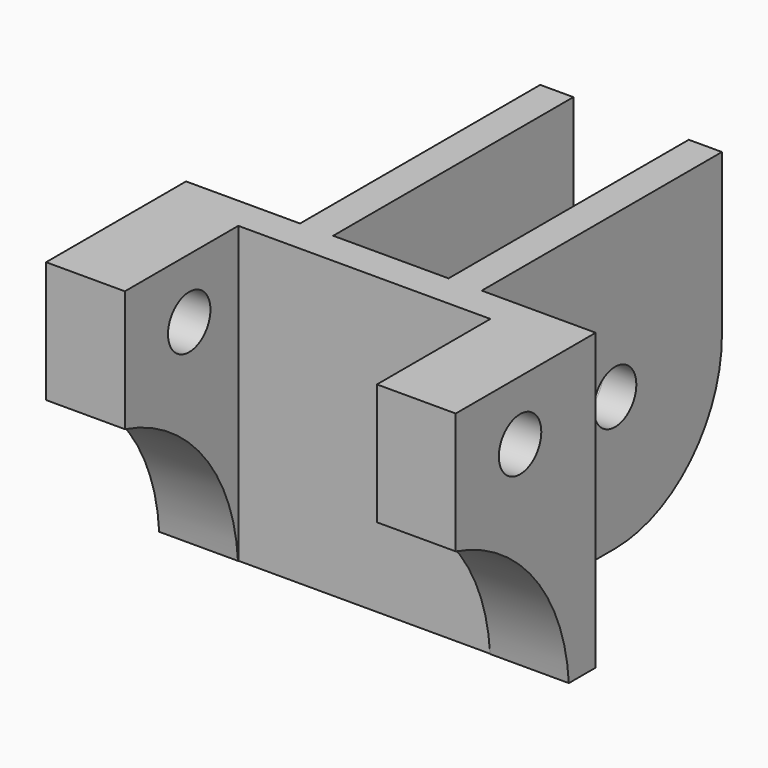
from build123d import *
from build123d import SkipClean  # not in build123d's __all__

# Parameters (mm, degrees)
F1_DEPTH  = 17.7784
F3_DEPTH  = 24.701
F4_R      = 1.6
F5_DEPTH  = 17.8292
F6_R      = 1.6
F7_DEPTH  = 24.701
F9_DEPTH  = 2
F10_R     = 3.2274
F10_R_2   = 1.6
F11_DEPTH = 0.5
F13_SIZE  = 0.49999
F14_R     = 8.052


# Not quite as in the source:
# - a fillet or chamfer is up to 0.001 mm smaller than in the source, because OpenCascade refuses the exact size


with BuildPart() as f1:
    # F0 (on Top) → F1 (new body)
    with BuildSketch(Plane.XY):
        Polygon((-3.4782, 5.7), (-3.4782, 23.8038), (-5.4782, 23.8038), (-5.4782, 5.7), (-12.35, 5.7), (-12.35, -4.85), (-7.6, -4.85), (-7.6, 3.7), (7.6, 3.7), (7.6, -4.85), (12.35, -4.85), (12.35, 5.7), (5.4782, 5.7), (5.4782, 23.8038), (3.4782, 23.8038), (3.4782, 5.7), align=None)
    extrude(amount=F1_DEPTH)

    # F2 (on face) → F3 (cut, through all)
    with BuildSketch(Plane.YZ.offset(12.35)):
        with BuildLine():
            Line((3.7, -12.353613347), (3.7, -0.741613347))
            ThreePointArc((3.7, -0.741613347), (1.3182353166, 6.3040448905), (-4.85, 10.4594))
            ThreePointArc((-4.85, 10.4594), (-19.420794702, 0.8031159196), (-7.912, -12.353613347))
            Line((-7.912, -12.353613347), (3.7, -12.353613347))
        make_face()
    extrude(amount=-F3_DEPTH, mode=Mode.SUBTRACT)

    # F4 (on face) → F5 (cut, through all)
    with BuildSketch(Plane.YZ.offset(5.4782)):
        with Locations((15.752, 8.0518)):
            Circle(F4_R)
    extrude(amount=-F5_DEPTH, mode=Mode.SUBTRACT)

    # F6 (on face) → F7 (cut, through all)
    with BuildSketch(Plane.YZ.offset(12.35)):
        with Locations((0, 14.1784)):
            Circle(F6_R)
    extrude(amount=-F7_DEPTH, mode=Mode.SUBTRACT)

    # F8 (on face) → F9 (cut)
    with BuildSketch(Plane(origin=(-12.35, 0, 0), x_dir=(0, -1, 0), z_dir=(-1, 0, 0))):
        Polygon((0, 17.4692965344), (-2.85, 15.8238482672), (-2.85, 12.5329517328), (0, 10.8875034656), (2.85, 12.5329517328), (2.85, 15.8238482672), align=None)
    extrude(amount=-F9_DEPTH, mode=Mode.SUBTRACT)



with BuildPart() as f11:
    # F10 (on face) → F11 (new body)
    with BuildSketch(Plane(origin=(3.4782, 0, 0), x_dir=(0, -1, 0), z_dir=(-1, 0, 0))):
        with Locations((-15.752, 8.0518)):
            Circle(F10_R)
        with Locations((-15.752, 8.0518)):
            Circle(F10_R_2, mode=Mode.SUBTRACT)
    extrude(amount=F11_DEPTH)


with BuildPart() as f1_1:
    add(f1.part, clean=False)

    with SkipClean():  # cleaning this boolean's faces spoils the solid; the shape is the same uncleaned
        add(f11.part)  # F12 merges F11
    # F12: F11 across plane
    with SkipClean():  # cleaning this boolean's faces spoils the solid; the shape is the same uncleaned
        add(f11.part.mirror(Plane.YZ), clean=False)

    # F13 (size 0.5 in the source; OpenCascade refuses exactly that, so slightly less here)
    f13_edges = [f1_1.edges().sort_by_distance(p)[0] for p in [
        (2.9782, 18.9794, 8.0518),
        (-2.9782, 18.9794, 8.0518),
    ]]
    chamfer(f13_edges, length=F13_SIZE)

    # F14
    f14_edges = [f1_1.edges().sort_by_distance(p)[0] for p in [
        (-4.4782, 23.8038, 0),
        (4.4782, 23.8038, 0),
    ]]
    fillet(f14_edges, radius=F14_R)


solid = f1_1.part
